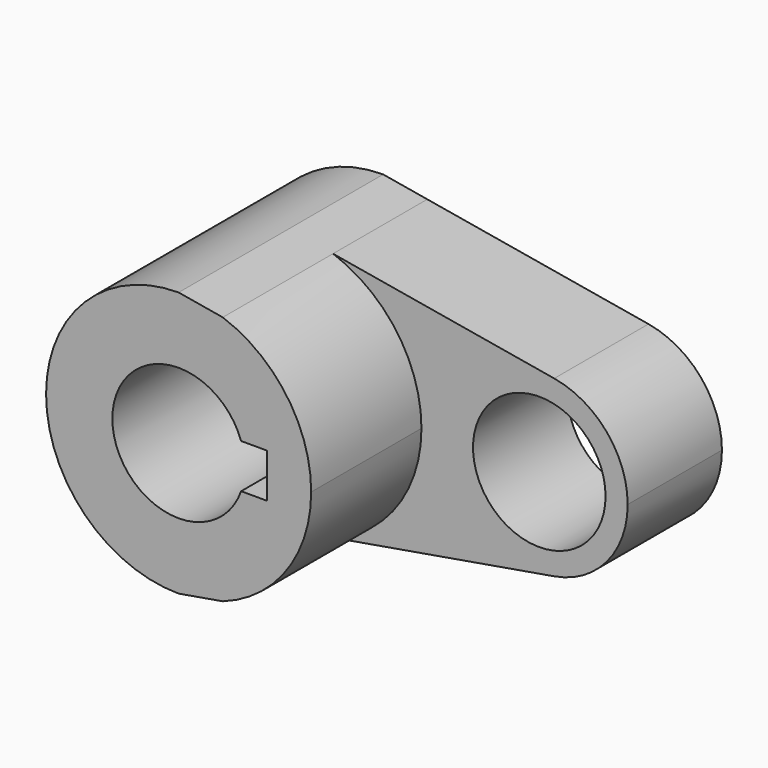
from build123d import *

# Parameters (mm, degrees)
F0_R     = 14.2875
F1_DEPTH = 25.4
F2_DEPTH = 25.4
F3_DEPTH = 55.118


with BuildPart() as f1:
    # F0 (on Front) → F1 (new body)
    with BuildSketch(Plane.XZ):
        with BuildLine():
            Line((9.5121844836, 26.9452959039), (0, 28.575))
            ThreePointArc((0, 28.575), (-28.575, 0), (0, -28.575))
            Line((0, -28.575), (9.5121844836, -26.9452959039))
            ThreePointArc((9.5121844836, -26.9452959039), (23.3274655355, -16.5033322905), (28.575, 0))
            ThreePointArc((28.575, 0), (23.3274655355, 16.5033322905), (9.5121844836, 26.9452959039))
        make_face()
        with BuildLine():
            ThreePointArc((-13.4703841816, 4.7625), (0, 14.2875), (13.4703841816, 4.7625))
            Line((13.4703841816, 4.7625), (19.05, 4.7625))
            Line((19.05, 4.7625), (19.05, -4.7625))
            Line((19.05, -4.7625), (13.4703841816, -4.7625))
            ThreePointArc((13.4703841816, -4.7625), (0, -14.2875), (-13.4703841816, -4.7625))
            Line((-13.4703841816, -4.7625), (-19.05, -4.7625))
            Line((-19.05, -4.7625), (-19.05, 4.7625))
            Line((-19.05, 4.7625), (-13.4703841816, 4.7625))
        make_face(mode=Mode.SUBTRACT)
        with BuildLine():
            Line((57.1919272622, 18.7764181619), (9.5121844836, 26.9452959039))
            ThreePointArc((9.5121844836, 26.9452959039), (23.3274655355, 16.5033322905), (28.575, 0))
            ThreePointArc((28.575, 0), (23.3274655355, -16.5033322905), (9.5121844836, -26.9452959039))
            Line((9.5121844836, -26.9452959039), (57.1919272622, -18.7764181619))
            ThreePointArc((57.1919272622, -18.7764181619), (34.925, 0), (57.1919272622, 18.7764181619))
        make_face()
        with BuildLine():
            ThreePointArc((73.025, 0), (68.5383952831, 12.2804730295), (57.1919272622, 18.7764181619))
            ThreePointArc((57.1919272622, 18.7764181619), (34.925, 0), (57.1919272622, -18.7764181619))
            ThreePointArc((57.1919272622, -18.7764181619), (68.5383952831, -12.2804730295), (73.025, 0))
        make_face()
        with Locations((53.975, 0)):
            Circle(F0_R, mode=Mode.SUBTRACT)
    extrude(amount=F1_DEPTH)

    # F0 (on Front) → F2 (join)
    with BuildSketch(Plane.XZ):
        with BuildLine():
            ThreePointArc((-13.4703841816, -4.7625), (-14.2875, 0), (-13.4703841816, 4.7625))
            Line((-13.4703841816, 4.7625), (-19.05, 4.7625))
            Line((-19.05, 4.7625), (-19.05, -4.7625))
            Line((-19.05, -4.7625), (-13.4703841816, -4.7625))
        make_face()
    extrude(amount=F2_DEPTH)

    # F0 (on Front) → F3 (join)
    with BuildSketch(Plane.XZ):
        with BuildLine():
            Line((9.5121844836, 26.9452959039), (0, 28.575))
            ThreePointArc((0, 28.575), (-28.575, 0), (0, -28.575))
            Line((0, -28.575), (9.5121844836, -26.9452959039))
            ThreePointArc((9.5121844836, -26.9452959039), (23.3274655355, -16.5033322905), (28.575, 0))
            ThreePointArc((28.575, 0), (23.3274655355, 16.5033322905), (9.5121844836, 26.9452959039))
        make_face()
        with BuildLine():
            ThreePointArc((-13.4703841816, 4.7625), (0, 14.2875), (13.4703841816, 4.7625))
            Line((13.4703841816, 4.7625), (19.05, 4.7625))
            Line((19.05, 4.7625), (19.05, -4.7625))
            Line((19.05, -4.7625), (13.4703841816, -4.7625))
            ThreePointArc((13.4703841816, -4.7625), (0, -14.2875), (-13.4703841816, -4.7625))
            Line((-13.4703841816, -4.7625), (-19.05, -4.7625))
            Line((-19.05, -4.7625), (-19.05, 4.7625))
            Line((-19.05, 4.7625), (-13.4703841816, 4.7625))
        make_face(mode=Mode.SUBTRACT)
        with BuildLine():
            ThreePointArc((-13.4703841816, -4.7625), (-14.2875, 0), (-13.4703841816, 4.7625))
            Line((-13.4703841816, 4.7625), (-19.05, 4.7625))
            Line((-19.05, 4.7625), (-19.05, -4.7625))
            Line((-19.05, -4.7625), (-13.4703841816, -4.7625))
        make_face()
    extrude(amount=F3_DEPTH)


solid = f1.part
